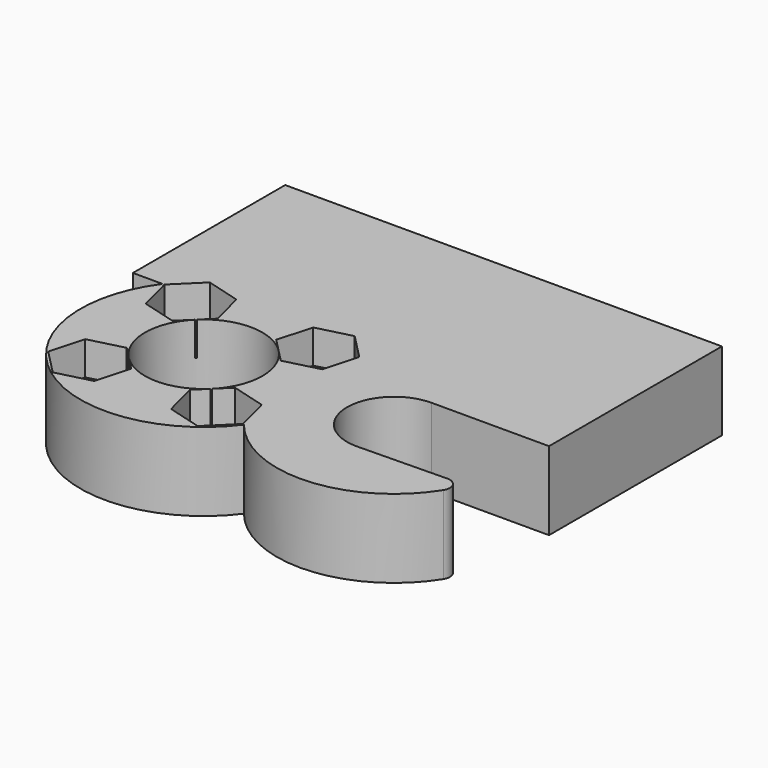
from build123d import *

# Parameters (mm, degrees)
F0_R     = 1.8
F0_R_2   = 5.25
F1_DEPTH = 7
F3_DEPTH = 3


# Not quite as in the source:
# - a feature names something its author has since deleted; it is built from what else it names


with BuildPart() as f1:
    # F0 (on Top) → F1 (new body)
    with BuildSketch(Plane.XY):
        with BuildLine():
            ThreePointArc((17, -4.2), (12.8000000278, 0.000483474), (17.000966948, 4.1999998887))
            Line((17.000966948, 4.1999998887), (27.4750051144, 4.1999998887))
            Line((27.4750051144, 4.1999998887), (27.4750051144, 23.499993239))
            Line((27.4750051144, 23.499993239), (-11.5249948856, 23.5))
            Line((-11.5249948856, 23.5), (-11.5249978328, 6.5))
            Line((-11.5249978328, 6.5), (-8.8741196746, 6.5))
            ThreePointArc((-8.8741196746, 6.5), (-6.5288626997, -8.8529064068), (8.8315992647, -6.5576561688))
            ThreePointArc((8.8315992647, -6.5576561688), (17.5981324789, -10.4579090901), (25.8628092229, -5.5835685434))
            ThreePointArc((25.8628092229, -5.5835685434), (25.8873322976, -4.5593941021), (24.9978561691, -4.051096075))
            Line((24.9978561691, -4.051096075), (17, -4.2))
        make_face()
        with Locations((-5.6568542495, -5.6568542495)):
            Circle(F0_R, mode=Mode.SUBTRACT)
        with Locations((5.6568542495, -5.6568542495)):
            Circle(F0_R, mode=Mode.SUBTRACT)
        with Locations((-5.6568542495, 5.6568542495)):
            Circle(F0_R, mode=Mode.SUBTRACT)
        Circle(F0_R_2, mode=Mode.SUBTRACT)
        with Locations((5.6568542495, 5.6568542495)):
            Circle(F0_R, mode=Mode.SUBTRACT)
    extrude(amount=-F1_DEPTH)

    # F2 (on face) → F3 (cut)
    with BuildSketch(Plane.XY):
        Polygon((-7.8783541444, -3.3878739609), (-8.7325987676, -6.4462394487), (-6.5110988727, -8.7152197373), (-3.4353543546, -7.9258345381), (-2.5811097314, -4.8674690503), (-4.8026096263, -2.5984887617), align=None)
        Polygon((3.3878739609, -7.8783541444), (6.4462394487, -8.7325987676), (8.7152197373, -6.5110988727), (7.9258345381, -3.4353543546), (4.8674690503, -2.5811097314), (2.5984887617, -4.8026096263), align=None)
        Polygon((7.8783541444, 3.3878739609), (8.7325987676, 6.4462394487), (6.5110988727, 8.7152197373), (3.4353543546, 7.9258345381), (2.5811097314, 4.8674690503), (4.8026096263, 2.5984887617), align=None)
        Polygon((-3.3878739609, 7.8783541444), (-6.4462394487, 8.7325987676), (-8.7152197373, 6.5110988727), (-7.9258345381, 3.4353543546), (-4.8674690503, 2.5811097314), (-2.5984887617, 4.8026096263), align=None)
    extrude(amount=-F3_DEPTH, mode=Mode.SUBTRACT)


solid = f1.part
